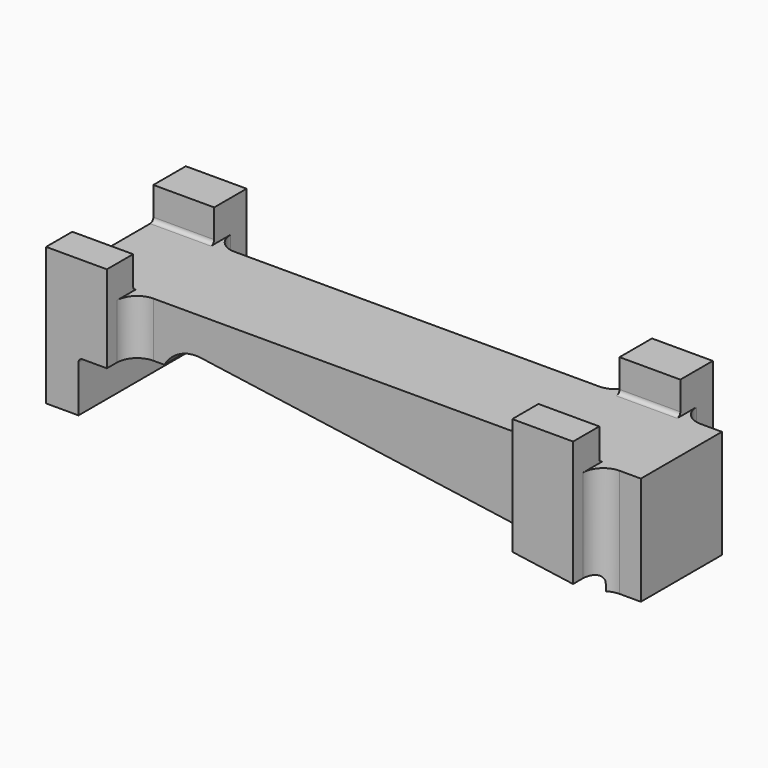
from build123d import *

# Parameters (mm, degrees)
F1_DEPTH  = 25
F3_DEPTH  = 130
F4_DEPTH  = 25
F5_R      = 5
F7_DEPTH  = 130
F8_DEPTH  = 25
F9_R      = 5
F10_R     = 1
F11_W     = 100
F11_H     = 10
F12_DEPTH = 35
F13_W     = 100
F13_H     = 8.0795794725
F14_DEPTH = 35
F15_R     = 5
F16_R     = 1


with BuildPart() as f1:
    # F0 (on Front) → F1 (new body)
    with BuildSketch(Plane.XZ):
        with BuildLine():
            ThreePointArc((-57.7942286341, 13.5), (-53.9433654568, 17.090109324), (-48.7430907909, 17.9118))
            Line((-48.7430907909, 17.9118), (50.034012295, 3.9804))
            ThreePointArc((50.034012295, 3.9804), (51.2644385711, 3.3117495349), (51.7546991374, 2))
            Line((51.7546991374, 2), (51.7546991374, 0.25))
            Line((51.7546991374, 0.25), (59.7546991374, 0.25))
            Line((59.7546991374, 0.25), (59.7546991374, 27))
            Line((59.7546991374, 27), (-80.5, 27))
            Line((-80.5, 27), (-80.5, 1))
            Line((-80.5, 1), (-72.5, 1))
            Line((-72.5, 1), (-72.5, 13.5))
            Line((-72.5, 13.5), (-57.7942286341, 13.5))
        make_face()
    extrude(amount=F1_DEPTH)

    # F2 (on face) → F3 (join)
    with BuildSketch(Plane(origin=(-80.5, 0, 0), x_dir=(0, -1, 0), z_dir=(-1, 0, 0))):
        Polygon((0, 1), (0, 27), (0, 35), (-10, 35), (-10, 1), align=None)
    extrude(amount=-F3_DEPTH)

    # F4 (cut): a face of the model
    f4_faces = [f1.faces().sort_by_distance(p)[0] for p in [
        (-23.2155862484, 0, 7.0978499246),
    ]]
    extrude(f4_faces, amount=-F4_DEPTH, mode=Mode.SUBTRACT)

    # F5
    f5_edges = [f1.edges().sort_by_distance(p)[0] for p in [
        (49.5, 0, 15.527858),
    ]]
    fillet(f5_edges, radius=F5_R)

    # F6 (on face) → F7 (join)
    with BuildSketch(Plane(origin=(-80.5, 0, 0), x_dir=(0, -1, 0), z_dir=(-1, 0, 0))):
        Polygon((25, 35), (25, 27), (25, 1), (33.0795794725, 1), (33.0795794725, 35), align=None)
    extrude(amount=-F7_DEPTH)

    # F8 (cut): a face of the model
    f8_faces = [f1.faces().sort_by_distance(p)[0] for p in [
        (-23.2155862484, -25, 7.0978499246),
    ]]
    extrude(f8_faces, amount=-F8_DEPTH, mode=Mode.SUBTRACT)

    # F9
    f9_edges = [f1.edges().sort_by_distance(p)[0] for p in [
        (49.5, -25, 15.527858),
    ]]
    fillet(f9_edges, radius=F9_R)

    # F10
    f10_edges = [f1.edges().sort_by_distance(p)[0] for p in [
        (-72.5, -11.53979, 13.5),
    ]]
    fillet(f10_edges, radius=F10_R)

    # F11 (on face) → F12 (cut)
    with BuildSketch(Plane.XY.offset(35)):
        with Locations((-15.5, 5)):
            Rectangle(F11_W, F11_H)
    extrude(amount=-F12_DEPTH, mode=Mode.SUBTRACT)

    # F13 (on face) → F14 (cut)
    with BuildSketch(Plane.XY.offset(35)):
        with Locations((-15.5, -29.0397897363)):
            Rectangle(F13_W, F13_H)
    extrude(amount=-F14_DEPTH, mode=Mode.SUBTRACT)

    # F15
    f15_edges = [f1.edges().sort_by_distance(p)[0] for p in [
        (-65.5, -25, 20.25),
        (-65.5, 0, 20.25),
        (34.5, 0, 16.585649),
        (34.5, -25, 16.585649),
    ]]
    fillet(f15_edges, radius=F15_R)

    # F16
    f16_edges = [f1.edges().sort_by_distance(p)[0] for p in [
        (42, -25, 27),
        (-73, -25, 27),
        (-73, 0, 27),
        (42, 0, 27),
    ]]
    fillet(f16_edges, radius=F16_R)


solid = f1.part
